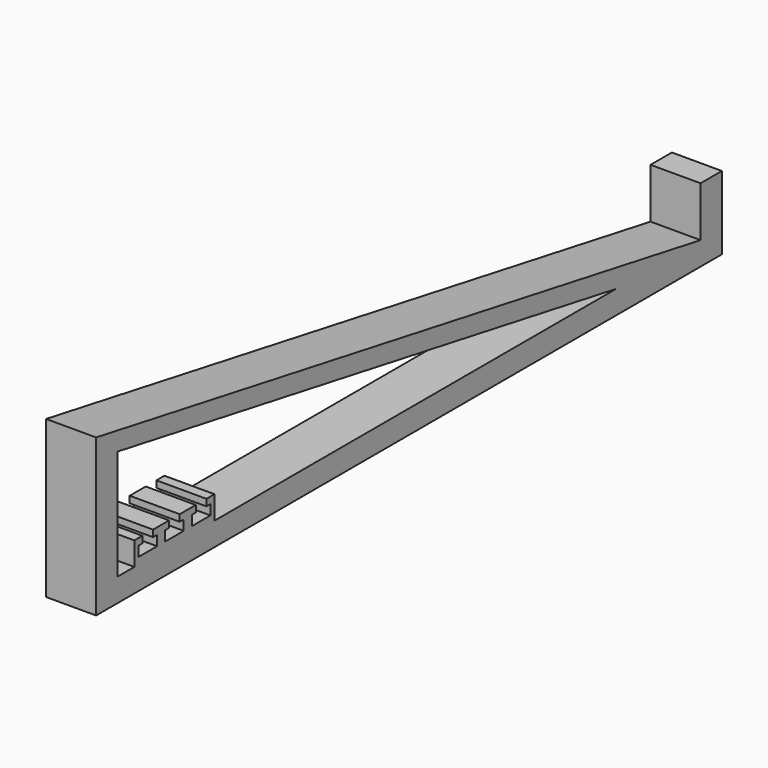
from build123d import *

# Parameters (mm, degrees)
F1_DEPTH = 15


# Not quite as in the source:
# - ends of sketch curves that miss each other by under 0.0002 mm in the source are joined


with BuildPart() as f1:
    # F0 (on Right) → F1 (new body)
    with BuildSketch(Plane.YZ):
        Polygon((57.2133171244, 7), (96.8499479096, 0), (96.8499479096, 22), (88.8499479096, 22), (88.8499479096, 7), align=None)
        Polygon((-129.6450851485, 0), (96.8499479096, 0), (57.2133171244, 7), (-93.3098772168, 7), (-103.3098761737, 7), (-113.3098740876, 7), (-123.3098730445, 7), (-129.6450851485, 7), align=None)
        Polygon((-129.6450851485, 40), (57.2133171244, 7), (88.8499479096, 7), (-137.6450851485, 47), (-137.6450851485, 0), (-129.6450851485, 0), (-129.6450851485, 7), align=None)
        Polygon((-123.3098730445, 14), (-123.3098730445, 7), (-113.3098740876, 7), (-113.3098730445, 14), (-116.3098730445, 14), (-116.3098730445, 12), (-114.8098730445, 12), (-114.8098730445, 9), (-121.8098730445, 9), (-121.8098730445, 12), (-120.3098730445, 12), (-120.3098730445, 14), align=None)
        Polygon((-113.3098740876, 7), (-103.3098761737, 7), (-103.3098751307, 14), (-106.3098751307, 14), (-106.3098751307, 12), (-104.8098751307, 12), (-104.8098751307, 9), (-111.8098751307, 9), (-111.8098751307, 12), (-110.3098751307, 12), (-110.3098751307, 14), (-113.3098751307, 14), align=None)
        Polygon((-103.3098761737, 7), (-93.3098772168, 7), (-93.3098772168, 14), (-96.3098772168, 14), (-96.3098772168, 12), (-94.8098772168, 12), (-94.8098772168, 9), (-101.8098772168, 9), (-101.8098772168, 12), (-100.3098772168, 12), (-100.3098772168, 14), (-103.3098772168, 14), align=None)
    extrude(amount=F1_DEPTH)


solid = f1.part
